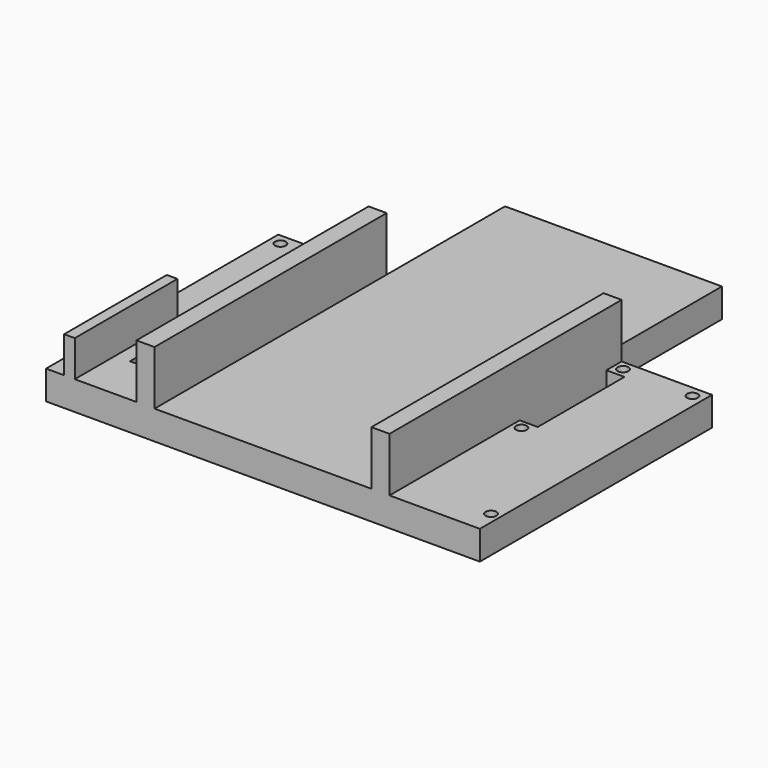
from build123d import *

# Parameters (mm, degrees)
F0_W     = 2.9425137265
F0_H     = 28.5
F0_W_2   = 6
F0_H_2   = 14.5
F0_W_3   = 4
F0_H_3   = 68
F0_W_4   = 1
F1_DEPTH = 5
F0_R     = 1.5
F0_W_5   = 5
F0_H_4   = 5.2732650286
F0_H_5   = 7
F0_W_6   = 17.0574862735
F0_H_6   = 5.2732627955
F2_DEPTH = 8
F3_DEPTH = 15
F4_DEPTH = 10
F5_D     = 3


# Not quite as in the source:
# - a feature names something its author has since deleted; it is built from what else it names


with BuildPart() as f1:
    # F0 (on Top) → F1 (new body)
    with BuildSketch(Plane.XY):
        with Locations((-55.0466683022, -35.8276315331)):
            Rectangle(F0_W, F0_H)
        Polygon((-53.5754114389, -21.5776315331), (-53.5754114389, -50.0776315331), (-36.5179251655, -50.0776315331), (-36.5179251655, -12.0776315331), (-41.5179251655, -12.0776315331), (-41.5179251655, 17.9223684669), (-56.5179251655, 17.9223684669), (-56.5179251655, -21.5776315331), align=None)
        with Locations((-46.5179251655, -35.8276315331)):
            Rectangle(F0_W_2, F0_H_2, mode=Mode.SUBTRACT)
        Polygon((-36.5179251655, -12.0776315331), (-36.5179251655, -50.0776315331), (-31.5179251655, -50.0776315331), (-31.5179251655, 17.9223684669), (-36.5179251655, 17.9223684669), align=None)
        with Locations((-29.5179251655, -16.0776315331)):
            Rectangle(F0_W_3, F0_H_3)
        with Locations((-27.0179251655, -16.0776315331)):
            Rectangle(F0_W_4, F0_H_3)
        Polygon((-31.5179251655, 23.1956334954), (-31.5179251655, 17.9223684669), (-27.5179251655, 17.9223684669), (-26.5179251655, 17.9223684669), (-26.5179251655, 58.8525284669), (-2.0179251655, 58.8525284669), (-1.5179251655, 58.8525284669), (-1.0179251655, 58.8525284669), (23.4820748345, 58.8525284669), (23.4820748345, 17.9223684669), (24.4820748345, 17.9223684669), (28.4820748345, 17.9223684669), (28.4820748345, 23.1956312623), (28.4820748345, 64.1257884669), (-31.5179251655, 64.1257884669), align=None)
        Polygon((-26.5179251655, 17.9223684669), (-26.5179251655, -50.0776315331), (-2.0179251655, -50.0776315331), (-2.0179251655, 58.8525284669), (-26.5179251655, 58.8525284669), align=None)
        Polygon((-2.0179251655, 58.8525284669), (-2.0179251655, -50.0776315331), (-1.0179251655, -50.0776315331), (-1.0179251655, 58.8525284669), (-1.5179251655, 58.8525284669), align=None)
        Polygon((28.4820748345, 17.9223684669), (28.4820748345, -50.0776315331), (33.4820748345, -50.0776315331), (33.4820748345, -17.0776315331), (33.4820748345, -12.0776315331), (33.4820748345, 17.9223684669), align=None)
        with Locations((26.4820748345, -16.0776315331)):
            Rectangle(F0_W_3, F0_H_3)
        Polygon((-1.0179251655, 58.8525284669), (-1.0179251655, -50.0776315331), (23.4820748345, -50.0776315331), (23.4820748345, 17.9223684669), (23.4820748345, 58.8525284669), align=None)
        Polygon((33.4820748345, -17.0776315331), (33.4820748345, -50.0776315331), (53.4820748345, -50.0776315331), (53.4820748345, 17.9223684669), (38.4820748345, 17.9223684669), (38.4820748345, -12.0776315331), (33.4820748345, -12.0776315331), align=None)
        with Locations((23.9820748345, -16.0776315331)):
            Rectangle(F0_W_4, F0_H_3)
    extrude(amount=-F1_DEPTH)

    # F0 (on Top) → F2 (join)
    with BuildSketch(Plane.XY):
        Polygon((-27.5179251655, -50.0776315331), (-31.5179251655, -50.0776315331), (-31.5179251655, -57.0776315331), (28.4820748345, -57.0776315331), (28.4820748345, -50.0776315331), (24.4820748345, -50.0776315331), (23.4820748345, -50.0776315331), (-1.0179251655, -50.0776315331), (-2.0179251655, -50.0776315331), (-26.5179251655, -50.0776315331), align=None)
        Polygon((-56.5179251655, -57.0776315331), (-56.5179251655, -50.0776315331), (-56.5179251655, -21.5776315331), (-56.5179251655, 17.9223684669), (-41.5179251655, 17.9223684669), (-36.5179251655, 17.9223684669), (-36.5179251655, 23.1956334954), (-61.5179251655, 23.1956334954), (-61.5179251655, -57.0776315331), align=None)
        with Locations((-59.0179251655, -50.0776315331)):
            Circle(F0_R, mode=Mode.SUBTRACT)
        with Locations((-58.5054894246, 20.1860783767)):
            Circle(F0_R, mode=Mode.SUBTRACT)
        Polygon((33.4820748345, -50.0776315331), (33.4820748345, -57.0776315331), (58.4820748345, -57.0776315331), (58.4820748345, 23.1956312623), (33.4820748345, 23.1956312623), (33.4820748345, 17.9223684669), (38.4820748345, 17.9223684669), (53.4820748345, 17.9223684669), (53.4820748345, -50.0776315331), align=None)
        with Locations((55.9820748345, -50.0776315331)):
            Circle(F0_R, mode=Mode.SUBTRACT)
        with Locations((55.4806331986, 20.1810636766)):
            Circle(F0_R, mode=Mode.SUBTRACT)
        with Locations((-34.0179251655, 20.5590009811)):
            Rectangle(F0_W_5, F0_H_4)
        with Locations((-55.0466683022, -53.5776315331)):
            Rectangle(F0_W, F0_H_5)
        with Locations((-45.0466683022, -53.5776315331)):
            Rectangle(F0_W_6, F0_H_5)
        with Locations((-34.0179251655, -53.5776315331)):
            Rectangle(F0_W_5, F0_H_5)
        with Locations((30.9820748345, -53.5776315331)):
            Rectangle(F0_W_5, F0_H_5)
        with Locations((-27.0179251655, -16.0776315331)):
            Rectangle(F0_W_4, F0_H_3)
        with Locations((23.9820748345, -16.0776315331)):
            Rectangle(F0_W_4, F0_H_3)
        Polygon((-2.0179251655, 58.8525284669), (-2.0179251655, -50.0776315331), (-1.0179251655, -50.0776315331), (-1.0179251655, 58.8525284669), (-1.5179251655, 58.8525284669), align=None)
        with Locations((30.9820748345, 20.5589998646)):
            Rectangle(F0_W_5, F0_H_6)
        with Locations((-34.0179251655, 20.5590009811)):
            Rectangle(F0_W_5, F0_H_4)
        Polygon((-31.5179251655, 23.1956334954), (-31.5179251655, 17.9223684669), (-27.5179251655, 17.9223684669), (-26.5179251655, 17.9223684669), (-26.5179251655, 58.8525284669), (-2.0179251655, 58.8525284669), (-1.5179251655, 58.8525284669), (-1.0179251655, 58.8525284669), (23.4820748345, 58.8525284669), (23.4820748345, 17.9223684669), (24.4820748345, 17.9223684669), (28.4820748345, 17.9223684669), (28.4820748345, 23.1956312623), (28.4820748345, 64.1257884669), (-31.5179251655, 64.1257884669), align=None)
        with Locations((30.9820748345, 20.5589998646)):
            Rectangle(F0_W_5, F0_H_6)
        with Locations((-34.0179251655, 20.5590009811)):
            Rectangle(F0_W_5, F0_H_4)
    extrude(amount=-F2_DEPTH)

    # F0 (on Top) → F3 (join)
    with BuildSketch(Plane.XY):
        Polygon((-36.5179251655, -12.0776315331), (-36.5179251655, -50.0776315331), (-31.5179251655, -50.0776315331), (-31.5179251655, 17.9223684669), (-36.5179251655, 17.9223684669), align=None)
        with Locations((-34.0179251655, -53.5776315331)):
            Rectangle(F0_W_5, F0_H_5)
        with Locations((-34.0179251655, 20.5590009811)):
            Rectangle(F0_W_5, F0_H_4)
        with Locations((30.9820748345, -53.5776315331)):
            Rectangle(F0_W_5, F0_H_5)
        Polygon((28.4820748345, 17.9223684669), (28.4820748345, -50.0776315331), (33.4820748345, -50.0776315331), (33.4820748345, -17.0776315331), (33.4820748345, -12.0776315331), (33.4820748345, 17.9223684669), align=None)
        with Locations((30.9820748345, 20.5589998646)):
            Rectangle(F0_W_5, F0_H_6)
    extrude(amount=F3_DEPTH)

    # F0 (on Top) → F4 (join)
    with BuildSketch(Plane.XY):
        with Locations((-55.0466683022, -35.8276315331)):
            Rectangle(F0_W, F0_H)
        with Locations((-55.0466683022, -53.5776315331)):
            Rectangle(F0_W, F0_H_5)
    extrude(amount=F4_DEPTH)

    # F5 (through all)
    with Locations(Plane.XY):
        with Locations((35.9820748345, 20.5589998646), (35.9820748345, -14.5776315331), (-39.0179251655, 20.5589998646), (-39.0179251655, -14.5776315331)):
            Hole(F5_D / 2)


solid = f1.part
